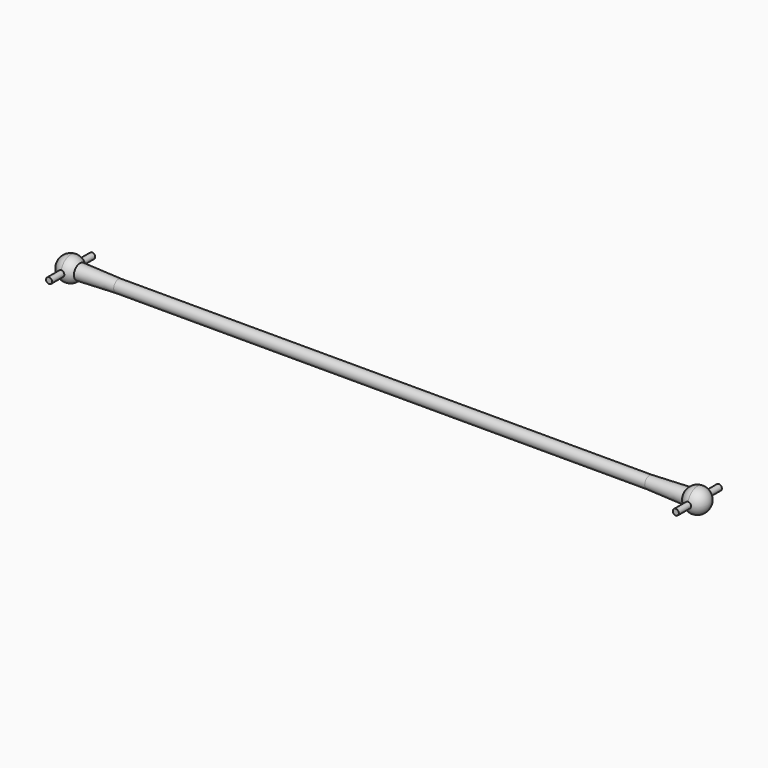
from build123d import *

# Parameters (mm, degrees)
F2_R     = 0.5
F3_DEPTH = 4.5
F4_R     = 0.5
F5_DEPTH = 4.5


# Not quite as in the source:
# - a feature names something its author has since deleted; it is built from what else it names


with BuildPart() as f1:
    # F0 (on Top) → F1 (revolve)
    with BuildSketch(Plane.XY):
        with BuildLine():
            Line((44.3736289605, -1), (50.8157129178, -1.2541521454))
            ThreePointArc((50.8157129178, -1.2541521454), (50.4873850625, -0.6648939444), (50.3736289605, 0))
            Line((50.3736289605, 0), (-50.3736289605, 0))
            ThreePointArc((-50.3736289605, 0), (-50.4873850625, -0.6648939444), (-50.8157129178, -1.2541521454))
            Line((-50.8157129178, -1.2541521454), (-44.3736289605, -1))
            Line((-44.3736289605, -1), (44.3736289605, -1))
        make_face()
        with BuildLine():
            ThreePointArc((-50.8157129178, -1.2541521454), (-50.4873850625, -0.6648939444), (-50.3736289605, 0))
            Line((-50.3736289605, 0), (-51.8736289605, 0))
            Line((-51.8736289605, 0), (-52.8736289605, 0))
            Line((-52.8736289605, 0), (-54.3736289605, 0))
            ThreePointArc((-54.3736289605, 0), (-53.7878425229, -1.4142135624), (-52.3736289605, -2))
            ThreePointArc((-52.3736289605, -2), (-51.5100041261, -1.8039268681), (-50.8157129178, -1.2541521454))
        make_face()
        with BuildLine():
            ThreePointArc((52.3736289605, -2), (53.7878425229, -1.4142135624), (54.3736289605, 0))
            Line((54.3736289605, 0), (52.8736289605, 0))
            Line((52.8736289605, 0), (52.3736289605, 0))
            Line((52.3736289605, 0), (51.8736289605, 0))
            Line((51.8736289605, 0), (50.3736289605, 0))
            ThreePointArc((50.3736289605, 0), (50.4873850625, -0.6648939444), (50.8157129178, -1.2541521454))
            ThreePointArc((50.8157129178, -1.2541521454), (51.5100041261, -1.8039268681), (52.3736289605, -2))
        make_face()
    revolve(axis=Axis((0, 0, 0), (1, 0, 0)))

    # F2 (on Front) → F3 (join, symmetric)
    with BuildSketch(Plane.XZ):
        with Locations((-52.3736289605, 0)):
            Circle(F2_R)
    extrude(amount=F3_DEPTH, both=True)

    # F4 (on Front) → F5 (join, symmetric)
    with BuildSketch(Plane.XZ):
        with Locations((52.3736289605, 0)):
            Circle(F4_R)
    extrude(amount=F5_DEPTH, both=True)


solid = f1.part
